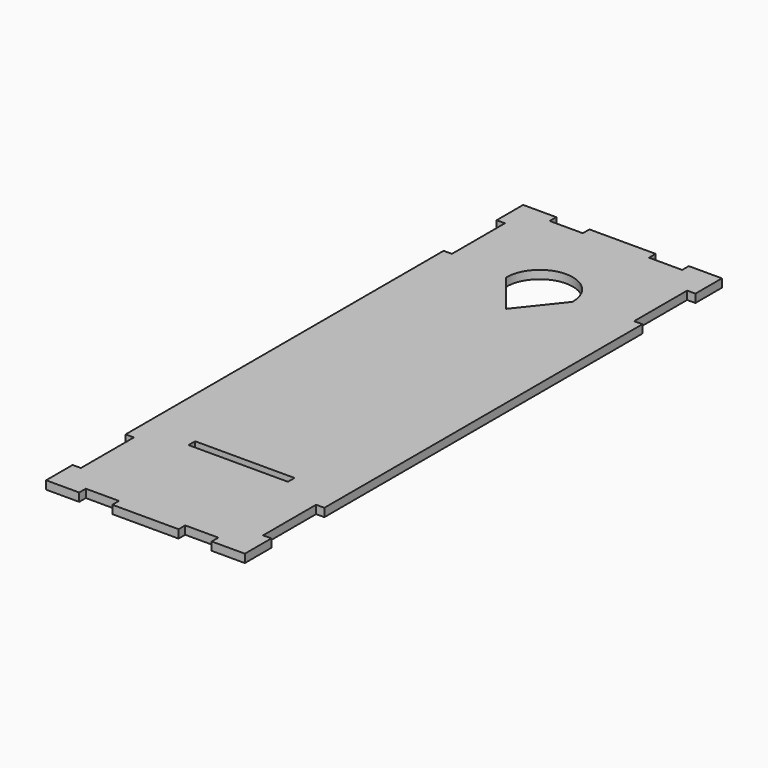
from build123d import *

# Parameters (mm, degrees)
F0_W             = 152.4
F0_H             = 457.2
F1_DEPTH         = 6.35
F2_W             = 25.4
F2_H             = 6.35
F3_DEPTH         = 6.351
F3_COPIES2_COUNT = 2
F3_COPIES3_COUNT = 2
F3_COPIES3_ANGLE = 90
F4_W             = 6.35
F4_H             = 50.8
F5_DEPTH         = 25.4
F6_W             = 76.2
F6_H             = 6.35
F7_DEPTH         = 25.4
F9_DEPTH         = 25.4


# Not quite as in the source:
# - a pattern or mirror of a feature is missing from the dataset's text; its kind, count and spacing are read off the source's solid


with BuildPart() as f1:
    # F0 (on Top) → F1 (new body)
    with BuildSketch(Plane.XY):
        Rectangle(F0_W, F0_H)
    extrude(amount=F1_DEPTH)

    # F2 (on face) → F3 (cut, through all)
    with BuildSketch(Plane.XY.offset(6.35)):
        with Locations((-38.1, 225.425)):
            Rectangle(F2_W, F2_H)
    f3 = extrude(amount=-F3_DEPTH, mode=Mode.SUBTRACT)

    # F3_copies: F3 across plane
    add(f3.mirror(Plane(origin=(0, 0, 0), x_dir=(0, 0, -1), z_dir=(0, -1, 0))), mode=Mode.SUBTRACT)

    # F3_copies1: F3 across plane
    add(f3.mirror(Plane(origin=(0, 0, 0), x_dir=(0, 0, 1), z_dir=(1, 0, 0))), mode=Mode.SUBTRACT)

    # F3_copies2: F3 ×2 about axis
    f3_copies2_axis = Axis((0, 0, 0), (0, 0, 1))
    for i in range(1, F3_COPIES2_COUNT):
        add(f3.rotate(f3_copies2_axis, i * 360 / F3_COPIES2_COUNT), mode=Mode.SUBTRACT)

    # F3_copies3: F3 ×2 about axis
    f3_copies3_axis = Axis((152.4, 0, 0), (0, 0, 1))
    for i in range(1, F3_COPIES3_COUNT):
        add(f3.rotate(f3_copies3_axis, i * F3_COPIES3_ANGLE / (F3_COPIES3_COUNT - 1)), mode=Mode.SUBTRACT)

    # F4 (on face) → F5 (cut)
    with BuildSketch(Plane.XY.offset(6.35)):
        with Locations((73.025, 177.8)):
            Rectangle(F4_W, F4_H)
        with Locations((73.025, -177.8)):
            Rectangle(F4_W, F4_H)
    f5 = extrude(amount=-F5_DEPTH, mode=Mode.SUBTRACT)

    # F5_copies: F5 across plane
    add(f5.mirror(Plane(origin=(0, 0, 0), x_dir=(0, 0, -1), z_dir=(-1, 0, 0))), mode=Mode.SUBTRACT)

    # F6 (on face) → F7 (cut)
    with BuildSketch(Plane.XY.offset(6.35)):
        with Locations((0, -136.525)):
            Rectangle(F6_W, F6_H)
    extrude(amount=-F7_DEPTH, mode=Mode.SUBTRACT)

    # F8 (on face) → F9 (cut)
    with BuildSketch(Plane.XY.offset(6.35)):
        with BuildLine():
            Line((0, 117.0066269137), (25.4, 148.9027270525))
            ThreePointArc((25.4, 148.9027270525), (0, 174.6158614811), (-25.4, 148.9027270525))
            Line((-25.4, 148.9027270525), (0, 117.0066269137))
        make_face()
    extrude(amount=-F9_DEPTH, mode=Mode.SUBTRACT)


solid = f1.part
